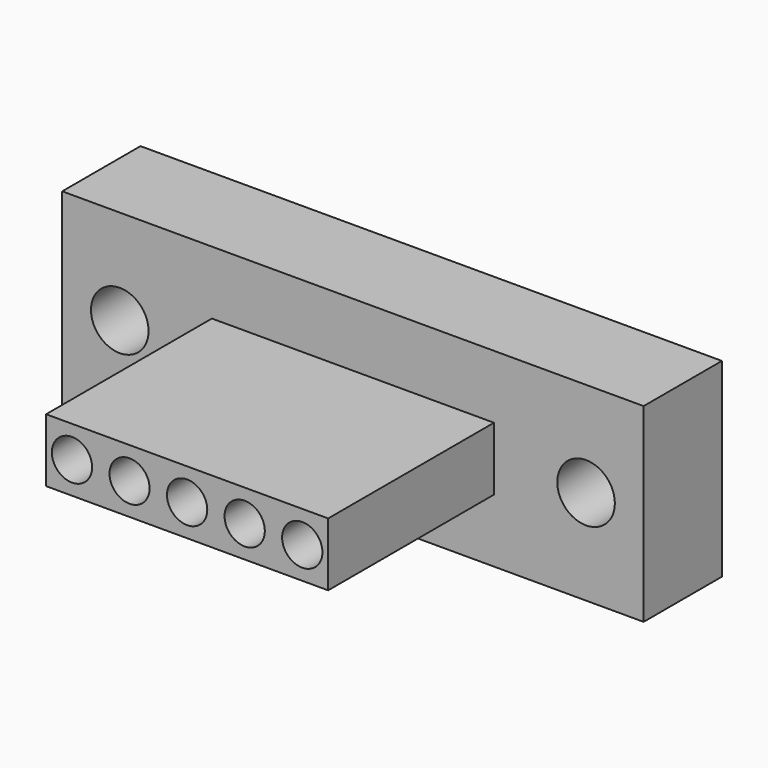
from build123d import *

# Parameters (mm, degrees)
F0_W     = 50.5
F0_H     = 16.5
F1_DEPTH = 8.5
F2_W     = 24.5
F2_H     = 5.5
F3_DEPTH = 18
F4_R     = 1.75
F4_R_2   = 1.7405151171
F5_DEPTH = 31.5
F6_R     = 2.5
F7_DEPTH = 8.5
F8_DEPTH = 25


# Not quite as in the source:
# - a feature names something its author has since deleted; it is built from what else it names


with BuildPart() as f1:
    # F0 (on Front) → F1 (new body)
    with BuildSketch(Plane.XZ):
        with Locations((-0.7638186216, 1.2478639662)):
            Rectangle(F0_W, F0_H)
    extrude(amount=F1_DEPTH)

    # F2 (on face) → F3 (join)
    with BuildSketch(Plane.XZ.offset(8.5)):
        with Locations((-0.7638186216, 1.2478639662)):
            Rectangle(F2_W, F2_H)
    extrude(amount=F3_DEPTH)

    # F4 (on face) → F5 (cut)
    with BuildSketch(Plane.XZ.offset(26.5)):
        with Locations((-10.7638186216, 1.2478639662)):
            Circle(F4_R)
        with Locations((-5.7638186216, 1.2478639662)):
            Circle(F4_R_2)
        with Locations((-0.7638186216, 1.2478639662)):
            Circle(F4_R)
        with Locations((4.2361813784, 1.2478639662)):
            Circle(F4_R)
        with Locations((9.2361813784, 1.2478639662)):
            Circle(F4_R)
    extrude(amount=-F5_DEPTH, mode=Mode.SUBTRACT)

    # F6 (on face) → F7 (cut)
    with BuildSketch(Plane.XZ.offset(8.5)):
        with Locations((-21.0138186216, 1.2478639662)):
            Circle(F6_R)
    extrude(amount=-F7_DEPTH, mode=Mode.SUBTRACT)

    # F6 (on face) → F8 (cut)
    with BuildSketch(Plane.XZ.offset(8.5)):
        with Locations((-21.0138186216, 1.2478639662)):
            Circle(F6_R)
        with Locations((19.4861813784, 1.2478639662)):
            Circle(F6_R)
    extrude(amount=-F8_DEPTH, mode=Mode.SUBTRACT)


solid = f1.part
